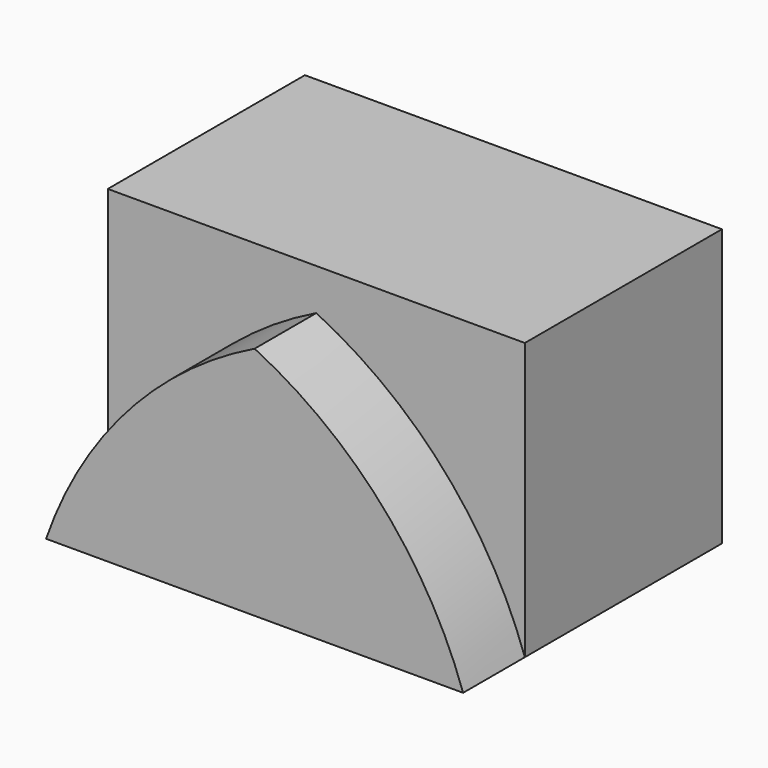
from build123d import *

# Parameters (mm, degrees)
F0_W        = 206.1633169651
F0_H        = 136.7557346821
F3_DEPTH    = 38.1348449737
F7_T1_DEPTH = 998.2832658749
F8_W        = 206.1633169651
F8_H        = 136.7557346821
F8_W_2      = 174.7721135616
F8_H_2      = 16.5176689625
F8_W_3      = 117.4946576357
F8_H_3      = 18.816370517
F2_W        = 206.1633169651
F2_H        = 136.7557346821
F9_DEPTH    = 121.7797268182


# Not quite as in the source:
# - a fillet or chamfer that OpenCascade refuses, or shapes differently, is made with other operations: its cross-section is extruded or revolved along the edge and cut away or added
# - the program builds the solid bodies; features that only make, move or delete a surface that nothing else refers to are left out


with BuildPart() as f3:
    # F0 (on Front) → F3 (new body)
    with BuildSketch(Plane.XZ):
        with Locations((1.0583624244, 0.0938400626)):
            Rectangle(F0_W, F0_H)
    extrude(amount=F3_DEPTH)

    # F7: fillet of radius 203.2 on 2 edges, made by hand

    # F7_s2 → F7_t1 (cut)
    with BuildSketch(Plane.XZ.offset(-480.0742104506)):
        with BuildLine():
            ThreePointArc((104.1400209069, -68.2840272784), (29.9847726477, 30.7886471902), (-87.8896632733, 68.4717074037))
            Line((-87.8896632733, 68.4717074037), (104.1400209069, 68.4717074037))
            Line((104.1400209069, 68.4717074037), (104.1400209069, -68.2840272784))
        make_face()
        with BuildLine():
            ThreePointArc((90.0063881221, 68.4717074037), (-27.868047799, 30.7886471902), (-102.0232960582, -68.2840272784))
            Line((-102.0232960582, -68.2840272784), (-102.0232960582, 68.4717074037))
            Line((-102.0232960582, 68.4717074037), (90.0063881221, 68.4717074037))
        make_face()
    extrude(amount=F7_T1_DEPTH, mode=Mode.SUBTRACT)

    # F8 (on face) + F2 (on face) → F9 (join)
    with BuildSketch(Plane.XZ):
        with Locations((1.0583624244, 0.0938400626)):
            Rectangle(F8_W, F8_H)
        with Locations((0, -32.6089076698)):
            Rectangle(F8_W_2, F8_H_2, mode=Mode.SUBTRACT)
        with Locations((10.9684318304, -3.3599911258)):
            Rectangle(F8_W_3, F8_H_3, mode=Mode.SUBTRACT)
    with BuildSketch(Plane.XZ):
        with Locations((1.0583624244, 0.0938400626)):
            Rectangle(F2_W, F2_H)
    extrude(amount=-F9_DEPTH)


solid = f3.part
